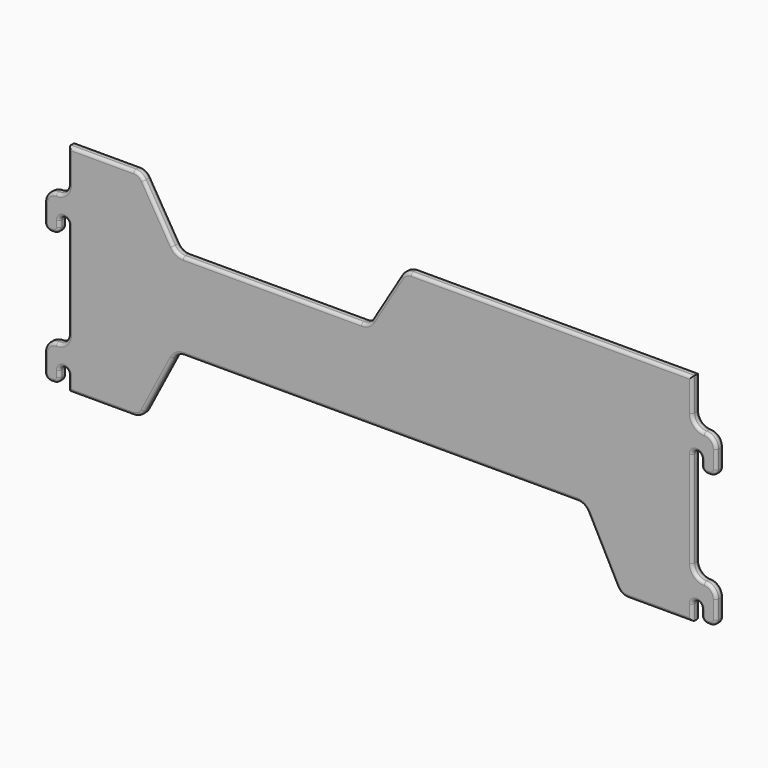
from build123d import *

# Parameters (mm, degrees)
F1_DEPTH      = 19.05
F2_R          = 25.39999
F3_T1_DEPTH   = 377.6375400722
F3_T3_DEPTH   = 832.8058394306
F3_T5_DEPTH   = 203.20001
F3_T7_DEPTH   = 12.7
F3_T9_DEPTH   = 6.35
F3_T11_DEPTH  = 38.1
F3_T13_DEPTH  = 1e-05
F3_T15_DEPTH  = 85.72501
F3_T17_DEPTH  = 38.1
F3_T19_DEPTH  = 12.7
F3_T21_DEPTH  = 47.625
F3_T23_DEPTH  = 1e-05
F3_T25_DEPTH  = 6.35
F3_T27_DEPTH  = 133.9390859232
F3_T29_DEPTH  = 152.8779197153
F3_T31_DEPTH  = 133.9390859232
F3_T33_DEPTH  = 152.8779197153
F3_T35_DEPTH  = 119.3437182012
F3_T37_DEPTH  = 153.8937700361
F3_T39_DEPTH  = 119.3437182012
F3_T41_DEPTH  = 611.0937700361
F3_T44_ANGLE  = 90
F3_T46_ANGLE  = 180
F3_T48_ANGLE  = 90
F3_T50_ANGLE  = 90
F3_T52_ANGLE  = 90
F3_T54_ANGLE  = 90
F3_T56_ANGLE  = 90
F3_T58_ANGLE  = 90
F3_T60_ANGLE  = 90
F3_T62_ANGLE  = 180
F3_T64_ANGLE  = 90
F3_T66_ANGLE  = 180
F3_T68_ANGLE  = 90
F3_T70_ANGLE  = 90
F3_T72_ANGLE  = 90
F3_T74_ANGLE  = 90
F3_T76_ANGLE  = 90
F3_T78_ANGLE  = 90
F3_T80_ANGLE  = 90
F3_T82_ANGLE  = 180
F3_T84_ANGLE  = 180
F3_T86_ANGLE  = 90
F3_T88_ANGLE  = 90
F3_T90_ANGLE  = 90
F3_T92_ANGLE  = 90
F3_T94_ANGLE  = 180
F3_T96_ANGLE  = 90
F3_T98_ANGLE  = 90
F3_T100_ANGLE = 90
F3_T102_ANGLE = 90
F3_T104_ANGLE = 180
F3_T106_ANGLE = 90
F3_T108_ANGLE = 90
F3_T110_ANGLE = 90
F3_T112_ANGLE = 90
F3_T114_ANGLE = 180
F3_T116_ANGLE = 90
F3_T118_ANGLE = 90
F3_T120_ANGLE = 90
F3_T122_ANGLE = 90
F3_T124_ANGLE = 62.4471884233
F3_T126_ANGLE = 62.4471884233
F3_T128_ANGLE = 62.4471884233
F3_T130_ANGLE = 62.4471884233
F3_T132_ANGLE = 59.0362434679
F3_T134_ANGLE = 59.0362434679
F3_T136_ANGLE = 59.0362434679
F3_T138_ANGLE = 59.0362434679
F3_T140_ANGLE = 62.4471884233
F3_T142_ANGLE = 62.4471884233
F3_T144_ANGLE = 62.4471884233
F3_T146_ANGLE = 62.4471884233
F3_T148_ANGLE = 59.0362434679
F3_T150_ANGLE = 59.0362434679
F3_T152_ANGLE = 59.0362434679
F3_T154_ANGLE = 59.0362434679


# Not quite as in the source:
# - a fillet or chamfer that OpenCascade refuses, or shapes differently, is made with other operations: its cross-section is extruded or revolved along the edge and cut away or added
# - a fillet or chamfer is up to 0.001 mm smaller than in the source, because OpenCascade refuses the exact size


with BuildPart() as f1:
    # F0 (on Front) → F1 (new body)
    with BuildSketch(Plane.XZ):
        Polygon((-508, 457.2), (-660.4, 457.2), (-660.4, 361.95), (-660.4, 311.15), (-660.4, 82.55), (-660.4, 31.75), (-660.4, 0), (-508, 0), (-431.8, 146.05), (431.8, 146.05), (508, 0), (660.4, 0), (660.4, 31.75), (660.4, 82.55), (660.4, 311.15), (660.4, 361.95), (660.4, 457.2), (50.8, 457.2), (-25.4, 330.2), (-431.8, 330.2), align=None)
        with BuildLine():
            Line((-660.4, 311.15), (-660.4, 361.95))
            Line((-660.4, 361.95), (-685.8, 361.95))
            ThreePointArc((-685.8, 361.95), (-703.7605122421, 354.5105122421), (-711.2, 336.55))
            Line((-711.2, 336.55), (-711.2, 298.45))
            ThreePointArc((-711.2, 298.45), (-707.4802561211, 289.4697438789), (-698.5, 285.75))
            Line((-698.5, 285.75), (-692.15, 285.75))
            ThreePointArc((-692.15, 285.75), (-683.1697438789, 289.4697438789), (-679.45, 298.45))
            Line((-679.45, 298.45), (-679.45, 311.15))
            ThreePointArc((-679.45, 311.15), (-669.925, 320.675), (-660.4, 311.15))
        make_face()
        with BuildLine():
            Line((-660.4, 31.75), (-660.4, 82.55))
            Line((-660.4, 82.55), (-685.8, 82.55))
            ThreePointArc((-685.8, 82.55), (-703.7605122421, 75.1105122421), (-711.2, 57.15))
            Line((-711.2, 57.15), (-711.2, 19.05))
            ThreePointArc((-711.2, 19.05), (-707.4802561211, 10.0697438789), (-698.5, 6.35))
            Line((-698.5, 6.35), (-692.15, 6.35))
            ThreePointArc((-692.15, 6.35), (-683.1697438789, 10.0697438789), (-679.45, 19.05))
            Line((-679.45, 19.05), (-679.45, 31.75))
            ThreePointArc((-679.45, 31.75), (-669.925, 41.275), (-660.4, 31.75))
        make_face()
        with BuildLine():
            Line((685.8, 361.95), (660.4, 361.95))
            Line((660.4, 361.95), (660.4, 311.15))
            ThreePointArc((660.4, 311.15), (669.925, 320.675), (679.45, 311.15))
            Line((679.45, 311.15), (679.45, 298.45))
            ThreePointArc((679.45, 298.45), (683.1697438789, 289.4697438789), (692.15, 285.75))
            Line((692.15, 285.75), (698.5, 285.75))
            ThreePointArc((698.5, 285.75), (707.4802561211, 289.4697438789), (711.2, 298.45))
            Line((711.2, 298.45), (711.2, 336.55))
            ThreePointArc((711.2, 336.55), (703.7605122421, 354.5105122421), (685.8, 361.95))
        make_face()
        with BuildLine():
            Line((685.8, 82.55), (660.4, 82.55))
            Line((660.4, 82.55), (660.4, 31.75))
            ThreePointArc((660.4, 31.75), (669.925, 41.275), (679.45, 31.75))
            Line((679.45, 31.75), (679.45, 19.05))
            ThreePointArc((679.45, 19.05), (683.1697438789, 10.0697438789), (692.15, 6.35))
            Line((692.15, 6.35), (698.5, 6.35))
            ThreePointArc((698.5, 6.35), (707.4802561211, 10.0697438789), (711.2, 19.05))
            Line((711.2, 19.05), (711.2, 57.15))
            ThreePointArc((711.2, 57.15), (703.7605122421, 75.1105122421), (685.8, 82.55))
        make_face()
    extrude(amount=-F1_DEPTH)

    # F2 (radius 25.4 in the source; OpenCascade refuses exactly that, so slightly less here)
    f2_edges = [f1.edges().sort_by_distance(p)[0] for p in [
        (-508, 9.525, 457.2),
        (-431.8, 9.525, 330.2),
        (50.8, 9.525, 457.2),
        (-25.4, 9.525, 330.2),
        (431.8, 9.525, 146.05),
        (508, 9.525, 0),
        (-431.8, 9.525, 146.05),
        (-508, 9.525, 0),
        (660.4, 9.525, 361.95),
        (660.4, 9.525, 82.55),
        (-660.4, 9.525, 82.55),
        (-660.4, 9.525, 361.95),
    ]]
    fillet(f2_edges, radius=F2_R)

    # F3: fillet of radius 6.35 on 8 edges, made by hand

    # F3_s2 → F3_t1 (cut)
    with BuildSketch(Plane.YZ.offset(-417.4187700361)):
        with BuildLine():
            ThreePointArc((0, 323.85), (1.8598719395, 328.3401280605), (6.35, 330.2))
            Line((6.35, 330.2), (0, 330.2))
            Line((0, 330.2), (0, 323.85))
        make_face()
        with BuildLine():
            ThreePointArc((19.05, 323.85), (17.1901280605, 328.3401280605), (12.7, 330.2))
            Line((12.7, 330.2), (19.05, 330.2))
            Line((19.05, 330.2), (19.05, 323.85))
        make_face()
    extrude(amount=F3_T1_DEPTH, mode=Mode.SUBTRACT)

    # F3_s4 → F3_t3 (cut)
    with BuildSketch(Plane.YZ.offset(-416.4029197153)):
        with BuildLine():
            ThreePointArc((0, 152.4), (1.8598719395, 147.9098719395), (6.35, 146.05))
            Line((6.35, 146.05), (0, 146.05))
            Line((0, 146.05), (0, 152.4))
        make_face()
        with BuildLine():
            ThreePointArc((19.05, 152.4), (17.1901280605, 147.9098719395), (12.7, 146.05))
            Line((12.7, 146.05), (19.05, 146.05))
            Line((19.05, 146.05), (19.05, 152.4))
        make_face()
    extrude(amount=F3_T3_DEPTH, mode=Mode.SUBTRACT)

    # F3_s6 → F3_t5 (cut)
    with BuildSketch(Plane.XY.offset(107.94999)):
        with BuildLine():
            ThreePointArc((-654.05, 19.05), (-658.5401280605, 17.1901280605), (-660.4, 12.7))
            Line((-660.4, 12.7), (-660.4, 19.05))
            Line((-660.4, 19.05), (-654.05, 19.05))
        make_face()
        with BuildLine():
            ThreePointArc((-654.05, 0), (-658.5401280605, 1.8598719395), (-660.4, 6.35))
            Line((-660.4, 6.35), (-660.4, 0))
            Line((-660.4, 0), (-654.05, 0))
        make_face()
        with BuildLine():
            ThreePointArc((654.05, 0), (658.5401280605, 1.8598719395), (660.4, 6.35))
            Line((660.4, 6.35), (660.4, 0))
            Line((660.4, 0), (654.05, 0))
        make_face()
        with BuildLine():
            ThreePointArc((654.05, 19.05), (658.5401280605, 17.1901280605), (660.4, 12.7))
            Line((660.4, 12.7), (660.4, 19.05))
            Line((660.4, 19.05), (654.05, 19.05))
        make_face()
    extrude(amount=F3_T5_DEPTH, mode=Mode.SUBTRACT)

    # F3_s8 → F3_t7 (cut)
    with BuildSketch(Plane.XY.offset(298.45)):
        with BuildLine():
            ThreePointArc((685.8, 19.05), (681.3098719395, 17.1901280605), (679.45, 12.7))
            Line((679.45, 12.7), (679.45, 19.05))
            Line((679.45, 19.05), (685.8, 19.05))
        make_face()
        with BuildLine():
            ThreePointArc((685.8, 0), (681.3098719395, 1.8598719395), (679.45, 6.35))
            Line((679.45, 6.35), (679.45, 0))
            Line((679.45, 0), (685.8, 0))
        make_face()
        with BuildLine():
            ThreePointArc((-685.8, 0), (-681.3098719395, 1.8598719395), (-679.45, 6.35))
            Line((-679.45, 6.35), (-679.45, 0))
            Line((-679.45, 0), (-685.8, 0))
        make_face()
        with BuildLine():
            ThreePointArc((-685.8, 19.05), (-681.3098719395, 17.1901280605), (-679.45, 12.7))
            Line((-679.45, 12.7), (-679.45, 19.05))
            Line((-679.45, 19.05), (-685.8, 19.05))
        make_face()
    extrude(amount=F3_T7_DEPTH, mode=Mode.SUBTRACT)

    # F3_s10 → F3_t9 (cut)
    with BuildSketch(Plane.YZ.offset(692.15)):
        with BuildLine():
            ThreePointArc((19.05, 292.1), (17.1901280605, 287.6098719395), (12.7, 285.75))
            Line((12.7, 285.75), (19.05, 285.75))
            Line((19.05, 285.75), (19.05, 292.1))
        make_face()
        with BuildLine():
            ThreePointArc((19.05, 12.7), (17.1901280605, 8.2098719395), (12.7, 6.35))
            Line((12.7, 6.35), (19.05, 6.35))
            Line((19.05, 6.35), (19.05, 12.7))
        make_face()
        with BuildLine():
            ThreePointArc((0, 292.1), (1.8598719395, 287.6098719395), (6.35, 285.75))
            Line((6.35, 285.75), (0, 285.75))
            Line((0, 285.75), (0, 292.1))
        make_face()
        with BuildLine():
            ThreePointArc((0, 12.7), (1.8598719395, 8.2098719395), (6.35, 6.35))
            Line((6.35, 6.35), (0, 6.35))
            Line((0, 6.35), (0, 12.7))
        make_face()
    extrude(amount=F3_T9_DEPTH, mode=Mode.SUBTRACT)

    # F3_s12 → F3_t11 (cut)
    with BuildSketch(Plane.XY.offset(298.45)):
        with BuildLine():
            ThreePointArc((704.85, 19.05), (709.3401280605, 17.1901280605), (711.2, 12.7))
            Line((711.2, 12.7), (711.2, 19.05))
            Line((711.2, 19.05), (704.85, 19.05))
        make_face()
        with BuildLine():
            ThreePointArc((704.85, 0), (709.3401280605, 1.8598719395), (711.2, 6.35))
            Line((711.2, 6.35), (711.2, 0))
            Line((711.2, 0), (704.85, 0))
        make_face()
        with BuildLine():
            ThreePointArc((-704.85, 0), (-709.3401280605, 1.8598719395), (-711.2, 6.35))
            Line((-711.2, 6.35), (-711.2, 0))
            Line((-711.2, 0), (-704.85, 0))
        make_face()
        with BuildLine():
            ThreePointArc((-704.85, 19.05), (-709.3401280605, 17.1901280605), (-711.2, 12.7))
            Line((-711.2, 12.7), (-711.2, 19.05))
            Line((-711.2, 19.05), (-704.85, 19.05))
        make_face()
    extrude(amount=F3_T11_DEPTH, mode=Mode.SUBTRACT)

    # F3_s14 → F3_t13 (cut)
    with BuildSketch(Plane.YZ.offset(685.79999)):
        with BuildLine():
            ThreePointArc((19.05, 355.6), (17.1901280605, 360.0901280605), (12.7, 361.95))
            Line((12.7, 361.95), (19.05, 361.95))
            Line((19.05, 361.95), (19.05, 355.6))
        make_face()
        with BuildLine():
            ThreePointArc((19.05, 76.2), (17.1901280605, 80.6901280605), (12.7, 82.55))
            Line((12.7, 82.55), (19.05, 82.55))
            Line((19.05, 82.55), (19.05, 76.2))
        make_face()
        with BuildLine():
            ThreePointArc((0, 355.6), (1.8598719395, 360.0901280605), (6.35, 361.95))
            Line((6.35, 361.95), (0, 361.95))
            Line((0, 361.95), (0, 355.6))
        make_face()
        with BuildLine():
            ThreePointArc((0, 76.2), (1.8598719395, 80.6901280605), (6.35, 82.55))
            Line((6.35, 82.55), (0, 82.55))
            Line((0, 82.55), (0, 76.2))
        make_face()
    extrude(amount=F3_T13_DEPTH, mode=Mode.SUBTRACT)

    # F3_s16 → F3_t15 (cut)
    with BuildSketch(Plane.XY.offset(387.34999)):
        with BuildLine():
            ThreePointArc((654.05, 19.05), (658.5401280605, 17.1901280605), (660.4, 12.7))
            Line((660.4, 12.7), (660.4, 19.05))
            Line((660.4, 19.05), (654.05, 19.05))
        make_face()
        with BuildLine():
            ThreePointArc((654.05, 0), (658.5401280605, 1.8598719395), (660.4, 6.35))
            Line((660.4, 6.35), (660.4, 0))
            Line((660.4, 0), (654.05, 0))
        make_face()
        with BuildLine():
            ThreePointArc((-654.05, 0), (-658.5401280605, 1.8598719395), (-660.4, 6.35))
            Line((-660.4, 6.35), (-660.4, 0))
            Line((-660.4, 0), (-654.05, 0))
        make_face()
        with BuildLine():
            ThreePointArc((-660.4, 12.7), (-658.5401280605, 17.1901280605), (-654.05, 19.05))
            Line((-654.05, 19.05), (-660.4, 19.05))
            Line((-660.4, 19.05), (-660.4, 12.7))
        make_face()
    extrude(amount=F3_T15_DEPTH, mode=Mode.SUBTRACT)

    # F3_s18 → F3_t17 (cut)
    with BuildSketch(Plane.XY.offset(19.05)):
        with BuildLine():
            ThreePointArc((704.85, 19.05), (709.3401280605, 17.1901280605), (711.2, 12.7))
            Line((711.2, 12.7), (711.2, 19.05))
            Line((711.2, 19.05), (704.85, 19.05))
        make_face()
        with BuildLine():
            ThreePointArc((704.85, 0), (709.3401280605, 1.8598719395), (711.2, 6.35))
            Line((711.2, 6.35), (711.2, 0))
            Line((711.2, 0), (704.85, 0))
        make_face()
        with BuildLine():
            ThreePointArc((-704.85, 0), (-709.3401280605, 1.8598719395), (-711.2, 6.35))
            Line((-711.2, 6.35), (-711.2, 0))
            Line((-711.2, 0), (-704.85, 0))
        make_face()
        with BuildLine():
            ThreePointArc((-704.85, 19.05), (-709.3401280605, 17.1901280605), (-711.2, 12.7))
            Line((-711.2, 12.7), (-711.2, 19.05))
            Line((-711.2, 19.05), (-704.85, 19.05))
        make_face()
    extrude(amount=F3_T17_DEPTH, mode=Mode.SUBTRACT)

    # F3_s20 → F3_t19 (cut)
    with BuildSketch(Plane.XY.offset(19.05)):
        with BuildLine():
            ThreePointArc((685.8, 19.05), (681.3098719395, 17.1901280605), (679.45, 12.7))
            Line((679.45, 12.7), (679.45, 19.05))
            Line((679.45, 19.05), (685.8, 19.05))
        make_face()
        with BuildLine():
            ThreePointArc((685.8, 0), (681.3098719395, 1.8598719395), (679.45, 6.35))
            Line((679.45, 6.35), (679.45, 0))
            Line((679.45, 0), (685.8, 0))
        make_face()
        with BuildLine():
            ThreePointArc((-685.8, 0), (-681.3098719395, 1.8598719395), (-679.45, 6.35))
            Line((-679.45, 6.35), (-679.45, 0))
            Line((-679.45, 0), (-685.8, 0))
        make_face()
        with BuildLine():
            ThreePointArc((-685.8, 19.05), (-681.3098719395, 17.1901280605), (-679.45, 12.7))
            Line((-679.45, 12.7), (-679.45, 19.05))
            Line((-679.45, 19.05), (-685.8, 19.05))
        make_face()
    extrude(amount=F3_T19_DEPTH, mode=Mode.SUBTRACT)

    # F3_s22 → F3_t21 (cut)
    with BuildSketch(Plane.XY.offset(-15.875)):
        with BuildLine():
            ThreePointArc((654.05, 19.05), (658.5401280605, 17.1901280605), (660.4, 12.7))
            Line((660.4, 12.7), (660.4, 19.05))
            Line((660.4, 19.05), (654.05, 19.05))
        make_face()
        with BuildLine():
            ThreePointArc((654.05, 0), (658.5401280605, 1.8598719395), (660.4, 6.35))
            Line((660.4, 6.35), (660.4, 0))
            Line((660.4, 0), (654.05, 0))
        make_face()
        with BuildLine():
            ThreePointArc((-654.05, 0), (-658.5401280605, 1.8598719395), (-660.4, 6.35))
            Line((-660.4, 6.35), (-660.4, 0))
            Line((-660.4, 0), (-654.05, 0))
        make_face()
        with BuildLine():
            ThreePointArc((-654.05, 19.05), (-658.5401280605, 17.1901280605), (-660.4, 12.7))
            Line((-660.4, 12.7), (-660.4, 19.05))
            Line((-660.4, 19.05), (-654.05, 19.05))
        make_face()
    extrude(amount=F3_T21_DEPTH, mode=Mode.SUBTRACT)

    # F3_s24 → F3_t23 (cut)
    with BuildSketch(Plane.YZ.offset(-685.8)):
        with BuildLine():
            ThreePointArc((0, 76.2), (1.8598719395, 80.6901280605), (6.35, 82.55))
            Line((6.35, 82.55), (0, 82.55))
            Line((0, 82.55), (0, 76.2))
        make_face()
        with BuildLine():
            ThreePointArc((0, 355.6), (1.8598719395, 360.0901280605), (6.35, 361.95))
            Line((6.35, 361.95), (0, 361.95))
            Line((0, 361.95), (0, 355.6))
        make_face()
        with BuildLine():
            ThreePointArc((19.05, 76.2), (17.1901280605, 80.6901280605), (12.7, 82.55))
            Line((12.7, 82.55), (19.05, 82.55))
            Line((19.05, 82.55), (19.05, 76.2))
        make_face()
        with BuildLine():
            ThreePointArc((19.05, 355.6), (17.1901280605, 360.0901280605), (12.7, 361.95))
            Line((12.7, 361.95), (19.05, 361.95))
            Line((19.05, 361.95), (19.05, 355.6))
        make_face()
    extrude(amount=F3_T23_DEPTH, mode=Mode.SUBTRACT)

    # F3_s26 → F3_t25 (cut)
    with BuildSketch(Plane.YZ.offset(-698.5)):
        with BuildLine():
            ThreePointArc((0, 12.7), (1.8598719395, 8.2098719395), (6.35, 6.35))
            Line((6.35, 6.35), (0, 6.35))
            Line((0, 6.35), (0, 12.7))
        make_face()
        with BuildLine():
            ThreePointArc((0, 292.1), (1.8598719395, 287.6098719395), (6.35, 285.75))
            Line((6.35, 285.75), (0, 285.75))
            Line((0, 285.75), (0, 292.1))
        make_face()
        with BuildLine():
            ThreePointArc((19.05, 12.7), (17.1901280605, 8.2098719395), (12.7, 6.35))
            Line((12.7, 6.35), (19.05, 6.35))
            Line((19.05, 6.35), (19.05, 12.7))
        make_face()
        with BuildLine():
            ThreePointArc((19.05, 292.1), (17.1901280605, 287.6098719395), (12.7, 285.75))
            Line((12.7, 285.75), (19.05, 285.75))
            Line((19.05, 285.75), (19.05, 292.1))
        make_face()
    extrude(amount=F3_T25_DEPTH, mode=Mode.SUBTRACT)

    # F3_s28 → F3_t27 (cut)
    with BuildSketch(Plane(origin=(39.6175597013, 0, -75.9336560942), x_dir=(0, 1, 0), z_dir=(0.4625660067, 0, -0.8865848462))):
        with BuildLine():
            ThreePointArc((19.05, 456.7351018521), (17.1901280605, 452.2449737915), (12.7, 450.3851018521))
            Line((12.7, 450.3851018521), (19.05, 450.3851018521))
            Line((19.05, 450.3851018521), (19.05, 456.7351018521))
        make_face()
        with BuildLine():
            ThreePointArc((0, 456.7351018521), (1.8598719395, 452.2449737915), (6.35, 450.3851018521))
            Line((6.35, 450.3851018521), (0, 450.3851018521))
            Line((0, 450.3851018521), (0, 456.7351018521))
        make_face()
    extrude(amount=F3_T27_DEPTH, mode=Mode.SUBTRACT)

    # F3_s30 → F3_t29 (cut)
    with BuildSketch(Plane.YZ.offset(523.3970802847)):
        with BuildLine():
            ThreePointArc((19.05, 6.35), (17.1901280605, 1.8598719395), (12.7, 0))
            Line((12.7, 0), (19.05, 0))
            Line((19.05, 0), (19.05, 6.35))
        make_face()
        with BuildLine():
            ThreePointArc((0, 6.35), (1.8598719395, 1.8598719395), (6.35, 0))
            Line((6.35, 0), (0, 0))
            Line((0, 0), (0, 6.35))
        make_face()
    extrude(amount=F3_T29_DEPTH, mode=Mode.SUBTRACT)

    # F3_s32 → F3_t31 (cut)
    with BuildSketch(Plane(origin=(-101.5732278172, 0, -194.682019983), x_dir=(0, 1, 0), z_dir=(0.4625660067, 0, 0.8865848462))):
        with BuildLine():
            ThreePointArc((19.05, 456.7351018521), (17.1901280605, 452.2449737915), (12.7, 450.3851018521))
            Line((12.7, 450.3851018521), (19.05, 450.3851018521))
            Line((19.05, 450.3851018521), (19.05, 456.7351018521))
        make_face()
        with BuildLine():
            ThreePointArc((0, 456.7351018521), (1.8598719395, 452.2449737915), (6.35, 450.3851018521))
            Line((6.35, 450.3851018521), (0, 450.3851018521))
            Line((0, 450.3851018521), (0, 456.7351018521))
        make_face()
    extrude(amount=F3_T31_DEPTH, mode=Mode.SUBTRACT)

    # F3_s34 → F3_t33 (cut)
    with BuildSketch(Plane.YZ.offset(-676.275)):
        with BuildLine():
            ThreePointArc((19.05, 6.35), (17.1901280605, 1.8598719395), (12.7, 0))
            Line((12.7, 0), (19.05, 0))
            Line((19.05, 0), (19.05, 6.35))
        make_face()
        with BuildLine():
            ThreePointArc((0, 6.35), (1.8598719395, 1.8598719395), (6.35, 0))
            Line((6.35, 0), (0, 0))
            Line((0, 0), (0, 6.35))
        make_face()
    extrude(amount=F3_T33_DEPTH, mode=Mode.SUBTRACT)

    # F3_s36 → F3_t35 (cut)
    with BuildSketch(Plane(origin=(-267.3755523625, 0, 445.6259206042), x_dir=(0, 1, 0), z_dir=(-0.5144957554, 0, 0.8574929257))):
        with BuildLine():
            ThreePointArc((19.05, 206.7289468805), (17.1901280605, 202.23881882), (12.7, 200.3789468805))
            Line((12.7, 200.3789468805), (19.05, 200.3789468805))
            Line((19.05, 200.3789468805), (19.05, 206.7289468805))
        make_face()
        with BuildLine():
            ThreePointArc((0, 206.7289468805), (1.8598719395, 202.23881882), (6.35, 200.3789468805))
            Line((6.35, 200.3789468805), (0, 200.3789468805))
            Line((0, 200.3789468805), (0, 206.7289468805))
        make_face()
    extrude(amount=F3_T35_DEPTH, mode=Mode.SUBTRACT)

    # F3_s38 → F3_t37 (cut)
    with BuildSketch(Plane.YZ.offset(-676.275)):
        with BuildLine():
            ThreePointArc((12.7, 457.2), (17.1901280605, 455.3401280605), (19.05, 450.85))
            Line((19.05, 450.85), (19.05, 457.2))
            Line((19.05, 457.2), (12.7, 457.2))
        make_face()
        with BuildLine():
            ThreePointArc((6.35, 457.2), (1.8598719395, 455.3401280605), (0, 450.85))
            Line((0, 450.85), (0, 457.2))
            Line((0, 457.2), (6.35, 457.2))
        make_face()
    extrude(amount=F3_T37_DEPTH, mode=Mode.SUBTRACT)

    # F3_s40 → F3_t39 (cut)
    with BuildSketch(Plane(origin=(207.7538594022, 0, 346.256432337), x_dir=(0, 1, 0), z_dir=(-0.5144957554, 0, -0.8574929257))):
        with BuildLine():
            ThreePointArc((19.05, -185.3168187553), (17.1901280605, -189.8069468158), (12.7, -191.6668187553))
            Line((12.7, -191.6668187553), (19.05, -191.6668187553))
            Line((19.05, -191.6668187553), (19.05, -185.3168187553))
        make_face()
        with BuildLine():
            ThreePointArc((0, -185.3168187553), (1.8598719395, -189.8069468158), (6.35, -191.6668187553))
            Line((6.35, -191.6668187553), (0, -191.6668187553))
            Line((0, -191.6668187553), (0, -185.3168187553))
        make_face()
    extrude(amount=F3_T39_DEPTH, mode=Mode.SUBTRACT)

    # F3_s42 → F3_t41 (cut)
    with BuildSketch(Plane.YZ.offset(65.1812299639)):
        with BuildLine():
            ThreePointArc((19.05, 450.85), (17.1901280605, 455.3401280605), (12.7, 457.2))
            Line((12.7, 457.2), (19.05, 457.2))
            Line((19.05, 457.2), (19.05, 450.85))
        make_face()
        with BuildLine():
            ThreePointArc((0, 450.85), (1.8598719395, 455.3401280605), (6.35, 457.2))
            Line((6.35, 457.2), (0, 457.2))
            Line((0, 457.2), (0, 450.85))
        make_face()
    extrude(amount=F3_T41_DEPTH, mode=Mode.SUBTRACT)

    # F3_s43 → F3_t44 (revolve, cut)
    with BuildSketch(Plane.YZ.offset(685.79999)):
        with BuildLine():
            ThreePointArc((19.05, 76.2), (17.1901280605, 80.6901280605), (12.7, 82.55))
            Line((12.7, 82.55), (19.05, 82.55))
            Line((19.05, 82.55), (19.05, 76.2))
        make_face()
    revolve(axis=Axis((685.79999, 19.05, 107.94999), (0, 1, 0)), revolution_arc=F3_T44_ANGLE, mode=Mode.SUBTRACT)

    # F3_s45 → F3_t46 (revolve, cut)
    with BuildSketch(Plane.XY.offset(311.15)):
        with BuildLine():
            ThreePointArc((654.05, 19.05), (658.5401280605, 17.1901280605), (660.4, 12.7))
            Line((660.4, 12.7), (660.4, 19.05))
            Line((660.4, 19.05), (654.05, 19.05))
        make_face()
    revolve(axis=Axis((669.925, 19.05, 311.15), (0, 1, 0)), revolution_arc=F3_T46_ANGLE, mode=Mode.SUBTRACT)

    # F3_s47 → F3_t48 (revolve, cut)
    with BuildSketch(Plane.XY.offset(298.45)):
        with BuildLine():
            ThreePointArc((685.8, 19.05), (681.3098719395, 17.1901280605), (679.45, 12.7))
            Line((679.45, 12.7), (679.45, 19.05))
            Line((679.45, 19.05), (685.8, 19.05))
        make_face()
    revolve(axis=Axis((692.15, 19.05, 298.45), (0, -1, 0)), revolution_arc=F3_T48_ANGLE, mode=Mode.SUBTRACT)

    # F3_s49 → F3_t50 (revolve, cut)
    with BuildSketch(Plane.YZ.offset(698.5)):
        with BuildLine():
            ThreePointArc((19.05, 292.1), (17.1901280605, 287.6098719395), (12.7, 285.75))
            Line((12.7, 285.75), (19.05, 285.75))
            Line((19.05, 285.75), (19.05, 292.1))
        make_face()
    revolve(axis=Axis((698.5, 19.05, 298.45), (0, -1, 0)), revolution_arc=F3_T50_ANGLE, mode=Mode.SUBTRACT)

    # F3_s51 → F3_t52 (revolve, cut)
    with BuildSketch(Plane.XY.offset(336.55)):
        with BuildLine():
            ThreePointArc((704.85, 19.05), (709.3401280605, 17.1901280605), (711.2, 12.7))
            Line((711.2, 12.7), (711.2, 19.05))
            Line((711.2, 19.05), (704.85, 19.05))
        make_face()
    revolve(axis=Axis((685.8, 19.05, 336.55), (0, -1, 0)), revolution_arc=F3_T52_ANGLE, mode=Mode.SUBTRACT)

    # F3_s53 → F3_t54 (revolve, cut)
    with BuildSketch(Plane.YZ.offset(685.79999)):
        with BuildLine():
            ThreePointArc((19.05, 355.6), (17.1901280605, 360.0901280605), (12.7, 361.95))
            Line((12.7, 361.95), (19.05, 361.95))
            Line((19.05, 361.95), (19.05, 355.6))
        make_face()
    revolve(axis=Axis((685.79999, 19.05, 387.34999), (0, 1, 0)), revolution_arc=F3_T54_ANGLE, mode=Mode.SUBTRACT)

    # F3_s55 → F3_t56 (revolve, cut)
    with BuildSketch(Plane.XY.offset(57.15)):
        with BuildLine():
            ThreePointArc((704.85, 19.05), (709.3401280605, 17.1901280605), (711.2, 12.7))
            Line((711.2, 12.7), (711.2, 19.05))
            Line((711.2, 19.05), (704.85, 19.05))
        make_face()
    revolve(axis=Axis((685.8, 19.05, 57.15), (0, -1, 0)), revolution_arc=F3_T56_ANGLE, mode=Mode.SUBTRACT)

    # F3_s57 → F3_t58 (revolve, cut)
    with BuildSketch(Plane.YZ.offset(698.5)):
        with BuildLine():
            ThreePointArc((19.05, 12.7), (17.1901280605, 8.2098719395), (12.7, 6.35))
            Line((12.7, 6.35), (19.05, 6.35))
            Line((19.05, 6.35), (19.05, 12.7))
        make_face()
    revolve(axis=Axis((698.5, 19.05, 19.05), (0, -1, 0)), revolution_arc=F3_T58_ANGLE, mode=Mode.SUBTRACT)

    # F3_s59 → F3_t60 (revolve, cut)
    with BuildSketch(Plane.XY.offset(19.05)):
        with BuildLine():
            ThreePointArc((685.8, 19.05), (681.3098719395, 17.1901280605), (679.45, 12.7))
            Line((679.45, 12.7), (679.45, 19.05))
            Line((679.45, 19.05), (685.8, 19.05))
        make_face()
    revolve(axis=Axis((692.15, 19.05, 19.05), (0, -1, 0)), revolution_arc=F3_T60_ANGLE, mode=Mode.SUBTRACT)

    # F3_s61 → F3_t62 (revolve, cut)
    with BuildSketch(Plane.XY.offset(31.75)):
        with BuildLine():
            ThreePointArc((654.05, 19.05), (658.5401280605, 17.1901280605), (660.4, 12.7))
            Line((660.4, 12.7), (660.4, 19.05))
            Line((660.4, 19.05), (654.05, 19.05))
        make_face()
    revolve(axis=Axis((669.925, 19.05, 31.75), (0, 1, 0)), revolution_arc=F3_T62_ANGLE, mode=Mode.SUBTRACT)

    # F3_s63 → F3_t64 (revolve, cut)
    with BuildSketch(Plane.YZ.offset(685.79999)):
        with BuildLine():
            ThreePointArc((0, 76.2), (1.8598719395, 80.6901280605), (6.35, 82.55))
            Line((6.35, 82.55), (0, 82.55))
            Line((0, 82.55), (0, 76.2))
        make_face()
    revolve(axis=Axis((685.79999, 0, 107.94999), (0, 1, 0)), revolution_arc=F3_T64_ANGLE, mode=Mode.SUBTRACT)

    # F3_s65 → F3_t66 (revolve, cut)
    with BuildSketch(Plane.XY.offset(311.15)):
        with BuildLine():
            ThreePointArc((654.05, 0), (658.5401280605, 1.8598719395), (660.4, 6.35))
            Line((660.4, 6.35), (660.4, 0))
            Line((660.4, 0), (654.05, 0))
        make_face()
    revolve(axis=Axis((669.925, 0, 311.15), (0, 1, 0)), revolution_arc=F3_T66_ANGLE, mode=Mode.SUBTRACT)

    # F3_s67 → F3_t68 (revolve, cut)
    with BuildSketch(Plane.XY.offset(298.45)):
        with BuildLine():
            ThreePointArc((685.8, 0), (681.3098719395, 1.8598719395), (679.45, 6.35))
            Line((679.45, 6.35), (679.45, 0))
            Line((679.45, 0), (685.8, 0))
        make_face()
    revolve(axis=Axis((692.15, 0, 298.45), (0, -1, 0)), revolution_arc=F3_T68_ANGLE, mode=Mode.SUBTRACT)

    # F3_s69 → F3_t70 (revolve, cut)
    with BuildSketch(Plane.YZ.offset(698.5)):
        with BuildLine():
            ThreePointArc((0, 292.1), (1.8598719395, 287.6098719395), (6.35, 285.75))
            Line((6.35, 285.75), (0, 285.75))
            Line((0, 285.75), (0, 292.1))
        make_face()
    revolve(axis=Axis((698.5, 0, 298.45), (0, -1, 0)), revolution_arc=F3_T70_ANGLE, mode=Mode.SUBTRACT)

    # F3_s71 → F3_t72 (revolve, cut)
    with BuildSketch(Plane.XY.offset(336.55)):
        with BuildLine():
            ThreePointArc((704.85, 0), (709.3401280605, 1.8598719395), (711.2, 6.35))
            Line((711.2, 6.35), (711.2, 0))
            Line((711.2, 0), (704.85, 0))
        make_face()
    revolve(axis=Axis((685.8, 0, 336.55), (0, -1, 0)), revolution_arc=F3_T72_ANGLE, mode=Mode.SUBTRACT)

    # F3_s73 → F3_t74 (revolve, cut)
    with BuildSketch(Plane.YZ.offset(685.79999)):
        with BuildLine():
            ThreePointArc((0, 355.6), (1.8598719395, 360.0901280605), (6.35, 361.95))
            Line((6.35, 361.95), (0, 361.95))
            Line((0, 361.95), (0, 355.6))
        make_face()
    revolve(axis=Axis((685.79999, 0, 387.34999), (0, 1, 0)), revolution_arc=F3_T74_ANGLE, mode=Mode.SUBTRACT)

    # F3_s75 → F3_t76 (revolve, cut)
    with BuildSketch(Plane.XY.offset(57.15)):
        with BuildLine():
            ThreePointArc((704.85, 0), (709.3401280605, 1.8598719395), (711.2, 6.35))
            Line((711.2, 6.35), (711.2, 0))
            Line((711.2, 0), (704.85, 0))
        make_face()
    revolve(axis=Axis((685.8, 0, 57.15), (0, -1, 0)), revolution_arc=F3_T76_ANGLE, mode=Mode.SUBTRACT)

    # F3_s77 → F3_t78 (revolve, cut)
    with BuildSketch(Plane.YZ.offset(698.5)):
        with BuildLine():
            ThreePointArc((0, 12.7), (1.8598719395, 8.2098719395), (6.35, 6.35))
            Line((6.35, 6.35), (0, 6.35))
            Line((0, 6.35), (0, 12.7))
        make_face()
    revolve(axis=Axis((698.5, 0, 19.05), (0, -1, 0)), revolution_arc=F3_T78_ANGLE, mode=Mode.SUBTRACT)

    # F3_s79 → F3_t80 (revolve, cut)
    with BuildSketch(Plane.XY.offset(19.05)):
        with BuildLine():
            ThreePointArc((685.8, 0), (681.3098719395, 1.8598719395), (679.45, 6.35))
            Line((679.45, 6.35), (679.45, 0))
            Line((679.45, 0), (685.8, 0))
        make_face()
    revolve(axis=Axis((692.15, 0, 19.05), (0, -1, 0)), revolution_arc=F3_T80_ANGLE, mode=Mode.SUBTRACT)

    # F3_s81 → F3_t82 (revolve, cut)
    with BuildSketch(Plane.XY.offset(31.75)):
        with BuildLine():
            ThreePointArc((654.05, 0), (658.5401280605, 1.8598719395), (660.4, 6.35))
            Line((660.4, 6.35), (660.4, 0))
            Line((660.4, 0), (654.05, 0))
        make_face()
    revolve(axis=Axis((669.925, 0, 31.75), (0, 1, 0)), revolution_arc=F3_T82_ANGLE, mode=Mode.SUBTRACT)

    # F3_s83 → F3_t84 (revolve, cut)
    with BuildSketch(Plane.XY.offset(311.15)):
        with BuildLine():
            ThreePointArc((-685.8, 0), (-681.3098719395, 1.8598719395), (-679.45, 6.35))
            Line((-679.45, 6.35), (-679.45, 0))
            Line((-679.45, 0), (-685.8, 0))
        make_face()
    revolve(axis=Axis((-669.925, 0, 311.15), (0, 1, 0)), revolution_arc=F3_T84_ANGLE, mode=Mode.SUBTRACT)

    # F3_s85 → F3_t86 (revolve, cut)
    with BuildSketch(Plane.XY.offset(107.94999)):
        with BuildLine():
            ThreePointArc((-654.05, 0), (-658.5401280605, 1.8598719395), (-660.4, 6.35))
            Line((-660.4, 6.35), (-660.4, 0))
            Line((-660.4, 0), (-654.05, 0))
        make_face()
    revolve(axis=Axis((-685.79999, 0, 107.94999), (0, 1, 0)), revolution_arc=F3_T86_ANGLE, mode=Mode.SUBTRACT)

    # F3_s87 → F3_t88 (revolve, cut)
    with BuildSketch(Plane.YZ.offset(-685.8)):
        with BuildLine():
            ThreePointArc((0, 76.2), (1.8598719395, 80.6901280605), (6.35, 82.55))
            Line((6.35, 82.55), (0, 82.55))
            Line((0, 82.55), (0, 76.2))
        make_face()
    revolve(axis=Axis((-685.8, 0, 57.15), (0, -1, 0)), revolution_arc=F3_T88_ANGLE, mode=Mode.SUBTRACT)

    # F3_s89 → F3_t90 (revolve, cut)
    with BuildSketch(Plane.XY.offset(19.05)):
        with BuildLine():
            ThreePointArc((-704.85, 0), (-709.3401280605, 1.8598719395), (-711.2, 6.35))
            Line((-711.2, 6.35), (-711.2, 0))
            Line((-711.2, 0), (-704.85, 0))
        make_face()
    revolve(axis=Axis((-698.5, 0, 19.05), (0, -1, 0)), revolution_arc=F3_T90_ANGLE, mode=Mode.SUBTRACT)

    # F3_s91 → F3_t92 (revolve, cut)
    with BuildSketch(Plane.YZ.offset(-692.15)):
        with BuildLine():
            ThreePointArc((0, 12.7), (1.8598719395, 8.2098719395), (6.35, 6.35))
            Line((6.35, 6.35), (0, 6.35))
            Line((0, 6.35), (0, 12.7))
        make_face()
    revolve(axis=Axis((-692.15, 0, 19.05), (0, -1, 0)), revolution_arc=F3_T92_ANGLE, mode=Mode.SUBTRACT)

    # F3_s93 → F3_t94 (revolve, cut)
    with BuildSketch(Plane.XY.offset(31.75)):
        with BuildLine():
            ThreePointArc((-685.8, 0), (-681.3098719395, 1.8598719395), (-679.45, 6.35))
            Line((-679.45, 6.35), (-679.45, 0))
            Line((-679.45, 0), (-685.8, 0))
        make_face()
    revolve(axis=Axis((-669.925, 0, 31.75), (0, 1, 0)), revolution_arc=F3_T94_ANGLE, mode=Mode.SUBTRACT)

    # F3_s95 → F3_t96 (revolve, cut)
    with BuildSketch(Plane.YZ.offset(-692.15)):
        with BuildLine():
            ThreePointArc((0, 292.1), (1.8598719395, 287.6098719395), (6.35, 285.75))
            Line((6.35, 285.75), (0, 285.75))
            Line((0, 285.75), (0, 292.1))
        make_face()
    revolve(axis=Axis((-692.15, 0, 298.45), (0, -1, 0)), revolution_arc=F3_T96_ANGLE, mode=Mode.SUBTRACT)

    # F3_s97 → F3_t98 (revolve, cut)
    with BuildSketch(Plane.XY.offset(298.45)):
        with BuildLine():
            ThreePointArc((-704.85, 0), (-709.3401280605, 1.8598719395), (-711.2, 6.35))
            Line((-711.2, 6.35), (-711.2, 0))
            Line((-711.2, 0), (-704.85, 0))
        make_face()
    revolve(axis=Axis((-698.5, 0, 298.45), (0, -1, 0)), revolution_arc=F3_T98_ANGLE, mode=Mode.SUBTRACT)

    # F3_s99 → F3_t100 (revolve, cut)
    with BuildSketch(Plane.YZ.offset(-685.8)):
        with BuildLine():
            ThreePointArc((0, 355.6), (1.8598719395, 360.0901280605), (6.35, 361.95))
            Line((6.35, 361.95), (0, 361.95))
            Line((0, 361.95), (0, 355.6))
        make_face()
    revolve(axis=Axis((-685.8, 0, 336.55), (0, -1, 0)), revolution_arc=F3_T100_ANGLE, mode=Mode.SUBTRACT)

    # F3_s101 → F3_t102 (revolve, cut)
    with BuildSketch(Plane.XY.offset(387.34999)):
        with BuildLine():
            ThreePointArc((-654.05, 0), (-658.5401280605, 1.8598719395), (-660.4, 6.35))
            Line((-660.4, 6.35), (-660.4, 0))
            Line((-660.4, 0), (-654.05, 0))
        make_face()
    revolve(axis=Axis((-685.79999, 0, 387.34999), (0, 1, 0)), revolution_arc=F3_T102_ANGLE, mode=Mode.SUBTRACT)

    # F3_s103 → F3_t104 (revolve, cut)
    with BuildSketch(Plane.XY.offset(311.15)):
        with BuildLine():
            ThreePointArc((-685.8, 19.05), (-681.3098719395, 17.1901280605), (-679.45, 12.7))
            Line((-679.45, 12.7), (-679.45, 19.05))
            Line((-679.45, 19.05), (-685.8, 19.05))
        make_face()
    revolve(axis=Axis((-669.925, 19.05, 311.15), (0, 1, 0)), revolution_arc=F3_T104_ANGLE, mode=Mode.SUBTRACT)

    # F3_s105 → F3_t106 (revolve, cut)
    with BuildSketch(Plane.XY.offset(107.94999)):
        with BuildLine():
            ThreePointArc((-654.05, 19.05), (-658.5401280605, 17.1901280605), (-660.4, 12.7))
            Line((-660.4, 12.7), (-660.4, 19.05))
            Line((-660.4, 19.05), (-654.05, 19.05))
        make_face()
    revolve(axis=Axis((-685.79999, 19.05, 107.94999), (0, 1, 0)), revolution_arc=F3_T106_ANGLE, mode=Mode.SUBTRACT)

    # F3_s107 → F3_t108 (revolve, cut)
    with BuildSketch(Plane.YZ.offset(-685.8)):
        with BuildLine():
            ThreePointArc((19.05, 76.2), (17.1901280605, 80.6901280605), (12.7, 82.55))
            Line((12.7, 82.55), (19.05, 82.55))
            Line((19.05, 82.55), (19.05, 76.2))
        make_face()
    revolve(axis=Axis((-685.8, 19.05, 57.15), (0, -1, 0)), revolution_arc=F3_T108_ANGLE, mode=Mode.SUBTRACT)

    # F3_s109 → F3_t110 (revolve, cut)
    with BuildSketch(Plane.XY.offset(19.05)):
        with BuildLine():
            ThreePointArc((-704.85, 19.05), (-709.3401280605, 17.1901280605), (-711.2, 12.7))
            Line((-711.2, 12.7), (-711.2, 19.05))
            Line((-711.2, 19.05), (-704.85, 19.05))
        make_face()
    revolve(axis=Axis((-698.5, 19.05, 19.05), (0, -1, 0)), revolution_arc=F3_T110_ANGLE, mode=Mode.SUBTRACT)

    # F3_s111 → F3_t112 (revolve, cut)
    with BuildSketch(Plane.YZ.offset(-692.15)):
        with BuildLine():
            ThreePointArc((19.05, 12.7), (17.1901280605, 8.2098719395), (12.7, 6.35))
            Line((12.7, 6.35), (19.05, 6.35))
            Line((19.05, 6.35), (19.05, 12.7))
        make_face()
    revolve(axis=Axis((-692.15, 19.05, 19.05), (0, -1, 0)), revolution_arc=F3_T112_ANGLE, mode=Mode.SUBTRACT)

    # F3_s113 → F3_t114 (revolve, cut)
    with BuildSketch(Plane.XY.offset(31.75)):
        with BuildLine():
            ThreePointArc((-685.8, 19.05), (-681.3098719395, 17.1901280605), (-679.45, 12.7))
            Line((-679.45, 12.7), (-679.45, 19.05))
            Line((-679.45, 19.05), (-685.8, 19.05))
        make_face()
    revolve(axis=Axis((-669.925, 19.05, 31.75), (0, 1, 0)), revolution_arc=F3_T114_ANGLE, mode=Mode.SUBTRACT)

    # F3_s115 → F3_t116 (revolve, cut)
    with BuildSketch(Plane.YZ.offset(-692.15)):
        with BuildLine():
            ThreePointArc((19.05, 292.1), (17.1901280605, 287.6098719395), (12.7, 285.75))
            Line((12.7, 285.75), (19.05, 285.75))
            Line((19.05, 285.75), (19.05, 292.1))
        make_face()
    revolve(axis=Axis((-692.15, 19.05, 298.45), (0, -1, 0)), revolution_arc=F3_T116_ANGLE, mode=Mode.SUBTRACT)

    # F3_s117 → F3_t118 (revolve, cut)
    with BuildSketch(Plane.XY.offset(298.45)):
        with BuildLine():
            ThreePointArc((-704.85, 19.05), (-709.3401280605, 17.1901280605), (-711.2, 12.7))
            Line((-711.2, 12.7), (-711.2, 19.05))
            Line((-711.2, 19.05), (-704.85, 19.05))
        make_face()
    revolve(axis=Axis((-698.5, 19.05, 298.45), (0, -1, 0)), revolution_arc=F3_T118_ANGLE, mode=Mode.SUBTRACT)

    # F3_s119 → F3_t120 (revolve, cut)
    with BuildSketch(Plane.YZ.offset(-685.8)):
        with BuildLine():
            ThreePointArc((19.05, 355.6), (17.1901280605, 360.0901280605), (12.7, 361.95))
            Line((12.7, 361.95), (19.05, 361.95))
            Line((19.05, 361.95), (19.05, 355.6))
        make_face()
    revolve(axis=Axis((-685.8, 19.05, 336.55), (0, -1, 0)), revolution_arc=F3_T120_ANGLE, mode=Mode.SUBTRACT)

    # F3_s121 → F3_t122 (revolve, cut)
    with BuildSketch(Plane.XY.offset(387.34999)):
        with BuildLine():
            ThreePointArc((-654.05, 19.05), (-658.5401280605, 17.1901280605), (-660.4, 12.7))
            Line((-660.4, 12.7), (-660.4, 19.05))
            Line((-660.4, 19.05), (-654.05, 19.05))
        make_face()
    revolve(axis=Axis((-685.79999, 19.05, 387.34999), (0, 1, 0)), revolution_arc=F3_T122_ANGLE, mode=Mode.SUBTRACT)

    # F3_s123 → F3_t124 (revolve, cut)
    with BuildSketch(Plane(origin=(-39.6175597013, 0, -75.9336560942), x_dir=(0, 1, 0), z_dir=(-0.4625660067, 0, -0.8865848462))):
        with BuildLine():
            ThreePointArc((19.05, -456.7351018521), (17.1901280605, -452.2449737915), (12.7, -450.3851018521))
            Line((12.7, -450.3851018521), (19.05, -450.3851018521))
            Line((19.05, -450.3851018521), (19.05, -456.7351018521))
        make_face()
    revolve(axis=Axis((-416.4029197153, 19.05, 120.65001), (0, 1, 0)), revolution_arc=F3_T124_ANGLE, mode=Mode.SUBTRACT)

    # F3_s125 → F3_t126 (revolve, cut)
    with BuildSketch(Plane.YZ.offset(416.4029197153)):
        with BuildLine():
            ThreePointArc((19.05, 152.4), (17.1901280605, 147.9098719395), (12.7, 146.05))
            Line((12.7, 146.05), (19.05, 146.05))
            Line((19.05, 146.05), (19.05, 152.4))
        make_face()
    revolve(axis=Axis((416.4029197153, 19.05, 120.65001), (0, 1, 0)), revolution_arc=F3_T126_ANGLE, mode=Mode.SUBTRACT)

    # F3_s127 → F3_t128 (revolve, cut)
    with BuildSketch(Plane(origin=(101.5732278172, 0, -194.682019983), x_dir=(0, 1, 0), z_dir=(-0.4625660067, 0, 0.8865848462))):
        with BuildLine():
            ThreePointArc((19.05, -456.7351018521), (17.1901280605, -452.2449737915), (12.7, -450.3851018521))
            Line((12.7, -450.3851018521), (19.05, -450.3851018521))
            Line((19.05, -450.3851018521), (19.05, -456.7351018521))
        make_face()
    revolve(axis=Axis((523.3970802847, 19.05, 25.39999), (0, -1, 0)), revolution_arc=F3_T128_ANGLE, mode=Mode.SUBTRACT)

    # F3_s129 → F3_t130 (revolve, cut)
    with BuildSketch(Plane.YZ.offset(-523.3970802847)):
        with BuildLine():
            ThreePointArc((19.05, 6.35), (17.1901280605, 1.8598719395), (12.7, 0))
            Line((12.7, 0), (19.05, 0))
            Line((19.05, 0), (19.05, 6.35))
        make_face()
    revolve(axis=Axis((-523.3970802847, 19.05, 25.39999), (0, -1, 0)), revolution_arc=F3_T130_ANGLE, mode=Mode.SUBTRACT)

    # F3_s131 → F3_t132 (revolve, cut)
    with BuildSketch(Plane(origin=(146.3520229507, 0, 243.9200382512), x_dir=(0, 1, 0), z_dir=(0.5144957554, 0, 0.8574929257))):
        with BuildLine():
            ThreePointArc((19.05, 185.3168187553), (17.1901280605, 189.8069468158), (12.7, 191.6668187553))
            Line((12.7, 191.6668187553), (19.05, 191.6668187553))
            Line((19.05, 191.6668187553), (19.05, 185.3168187553))
        make_face()
    revolve(axis=Axis((-39.7812299639, 19.05, 355.59999), (0, 1, 0)), revolution_arc=F3_T132_ANGLE, mode=Mode.SUBTRACT)

    # F3_s133 → F3_t134 (revolve, cut)
    with BuildSketch(Plane.YZ.offset(-417.4187700361)):
        with BuildLine():
            ThreePointArc((19.05, 323.85), (17.1901280605, 328.3401280605), (12.7, 330.2))
            Line((12.7, 330.2), (19.05, 330.2))
            Line((19.05, 330.2), (19.05, 323.85))
        make_face()
    revolve(axis=Axis((-417.4187700361, 19.05, 355.59999), (0, 1, 0)), revolution_arc=F3_T134_ANGLE, mode=Mode.SUBTRACT)

    # F3_s135 → F3_t136 (revolve, cut)
    with BuildSketch(Plane.YZ.offset(-522.3812299639)):
        with BuildLine():
            ThreePointArc((12.7, 457.2), (17.1901280605, 455.3401280605), (19.05, 450.85))
            Line((19.05, 450.85), (19.05, 457.2))
            Line((19.05, 457.2), (12.7, 457.2))
        make_face()
    revolve(axis=Axis((-522.3812299639, 19.05, 431.80001), (0, 1, 0)), revolution_arc=F3_T136_ANGLE, mode=Mode.SUBTRACT)

    # F3_s137 → F3_t138 (revolve, cut)
    with BuildSketch(Plane.YZ.offset(65.1812299639)):
        with BuildLine():
            ThreePointArc((19.05, 450.85), (17.1901280605, 455.3401280605), (12.7, 457.2))
            Line((12.7, 457.2), (19.05, 457.2))
            Line((19.05, 457.2), (19.05, 450.85))
        make_face()
    revolve(axis=Axis((65.1812299639, 19.05, 431.80001), (0, -1, 0)), revolution_arc=F3_T138_ANGLE, mode=Mode.SUBTRACT)

    # F3_s139 → F3_t140 (revolve, cut)
    with BuildSketch(Plane(origin=(-39.6175597013, 0, -75.9336560942), x_dir=(0, 1, 0), z_dir=(-0.4625660067, 0, -0.8865848462))):
        with BuildLine():
            ThreePointArc((0, -456.7351018521), (1.8598719395, -452.2449737915), (6.35, -450.3851018521))
            Line((6.35, -450.3851018521), (0, -450.3851018521))
            Line((0, -450.3851018521), (0, -456.7351018521))
        make_face()
    revolve(axis=Axis((-416.4029197153, 0, 120.65001), (0, 1, 0)), revolution_arc=F3_T140_ANGLE, mode=Mode.SUBTRACT)

    # F3_s141 → F3_t142 (revolve, cut)
    with BuildSketch(Plane.YZ.offset(416.4029197153)):
        with BuildLine():
            ThreePointArc((0, 152.4), (1.8598719395, 147.9098719395), (6.35, 146.05))
            Line((6.35, 146.05), (0, 146.05))
            Line((0, 146.05), (0, 152.4))
        make_face()
    revolve(axis=Axis((416.4029197153, 0, 120.65001), (0, 1, 0)), revolution_arc=F3_T142_ANGLE, mode=Mode.SUBTRACT)

    # F3_s143 → F3_t144 (revolve, cut)
    with BuildSketch(Plane(origin=(101.5732278172, 0, -194.682019983), x_dir=(0, 1, 0), z_dir=(-0.4625660067, 0, 0.8865848462))):
        with BuildLine():
            ThreePointArc((0, -456.7351018521), (1.8598719395, -452.2449737915), (6.35, -450.3851018521))
            Line((6.35, -450.3851018521), (0, -450.3851018521))
            Line((0, -450.3851018521), (0, -456.7351018521))
        make_face()
    revolve(axis=Axis((523.3970802847, 0, 25.39999), (0, -1, 0)), revolution_arc=F3_T144_ANGLE, mode=Mode.SUBTRACT)

    # F3_s145 → F3_t146 (revolve, cut)
    with BuildSketch(Plane.YZ.offset(-523.3970802847)):
        with BuildLine():
            ThreePointArc((0, 6.35), (1.8598719395, 1.8598719395), (6.35, 0))
            Line((6.35, 0), (0, 0))
            Line((0, 0), (0, 6.35))
        make_face()
    revolve(axis=Axis((-523.3970802847, 0, 25.39999), (0, -1, 0)), revolution_arc=F3_T146_ANGLE, mode=Mode.SUBTRACT)

    # F3_s147 → F3_t148 (revolve, cut)
    with BuildSketch(Plane(origin=(146.3520229507, 0, 243.9200382512), x_dir=(0, 1, 0), z_dir=(0.5144957554, 0, 0.8574929257))):
        with BuildLine():
            ThreePointArc((0, 185.3168187553), (1.8598719395, 189.8069468158), (6.35, 191.6668187553))
            Line((6.35, 191.6668187553), (0, 191.6668187553))
            Line((0, 191.6668187553), (0, 185.3168187553))
        make_face()
    revolve(axis=Axis((-39.7812299639, 0, 355.59999), (0, 1, 0)), revolution_arc=F3_T148_ANGLE, mode=Mode.SUBTRACT)

    # F3_s149 → F3_t150 (revolve, cut)
    with BuildSketch(Plane.YZ.offset(-417.4187700361)):
        with BuildLine():
            ThreePointArc((0, 323.85), (1.8598719395, 328.3401280605), (6.35, 330.2))
            Line((6.35, 330.2), (0, 330.2))
            Line((0, 330.2), (0, 323.85))
        make_face()
    revolve(axis=Axis((-417.4187700361, 0, 355.59999), (0, 1, 0)), revolution_arc=F3_T150_ANGLE, mode=Mode.SUBTRACT)

    # F3_s151 → F3_t152 (revolve, cut)
    with BuildSketch(Plane.YZ.offset(-522.3812299639)):
        with BuildLine():
            ThreePointArc((0, 450.85), (1.8598719395, 455.3401280605), (6.35, 457.2))
            Line((6.35, 457.2), (0, 457.2))
            Line((0, 457.2), (0, 450.85))
        make_face()
    revolve(axis=Axis((-522.3812299639, 0, 431.80001), (0, 1, 0)), revolution_arc=F3_T152_ANGLE, mode=Mode.SUBTRACT)

    # F3_s153 → F3_t154 (revolve, cut)
    with BuildSketch(Plane.YZ.offset(65.1812299639)):
        with BuildLine():
            ThreePointArc((0, 450.85), (1.8598719395, 455.3401280605), (6.35, 457.2))
            Line((6.35, 457.2), (0, 457.2))
            Line((0, 457.2), (0, 450.85))
        make_face()
    revolve(axis=Axis((65.1812299639, 0, 431.80001), (0, -1, 0)), revolution_arc=F3_T154_ANGLE, mode=Mode.SUBTRACT)


solid = f1.part
